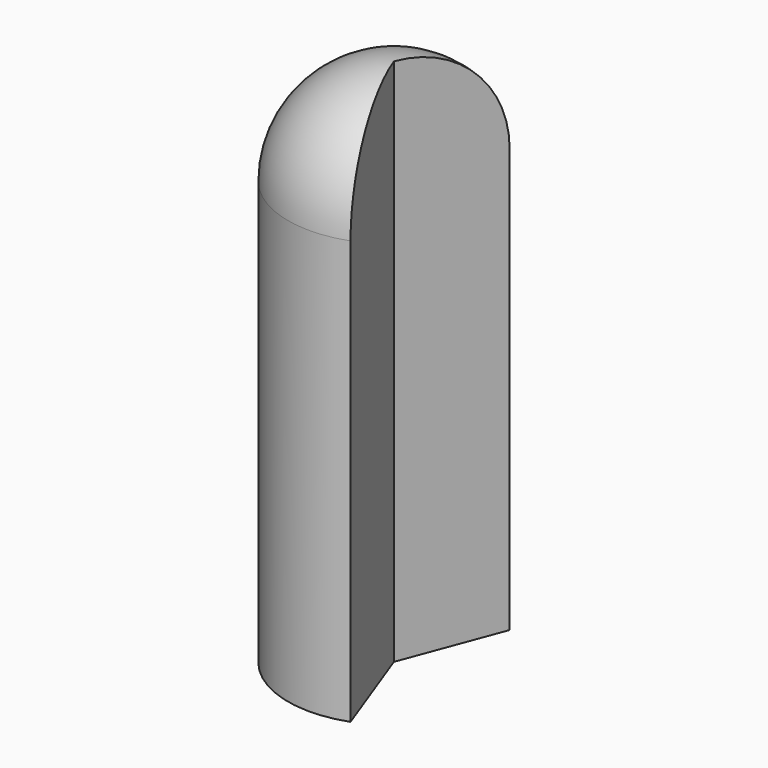
from build123d import *

# Parameters (mm, degrees)
F1_ANGLE_BACK = 110
F1_ANGLE      = 220


# Not quite as in the source:
# - a feature of the source that left no trace in its solid (it failed there, or was rolled back) is left out


with BuildPart() as f1:
    # F0 (on Front) → F1 (revolve)
    with BuildSketch(Plane.XZ, mode=Mode.PRIVATE) as f1_sk:
        with BuildLine():
            ThreePointArc((0, 253.6952), (-35.9210244843, 238.8162244843), (-50.8, 202.8952))
            Line((-50.8, 202.8952), (-50.8, -0.3048))
            Line((-50.8, -0.3048), (0, 0))
            Line((0, 0), (0, 202.8952))
            Line((0, 202.8952), (0, 253.6952))
        make_face()
    revolve(f1_sk.sketch.rotate(Axis((0, 0, 126.8476), (0, 0, -1)), -F1_ANGLE_BACK), axis=Axis((0, 0, 126.8476), (0, 0, -1)), revolution_arc=F1_ANGLE)


solid = f1.part
